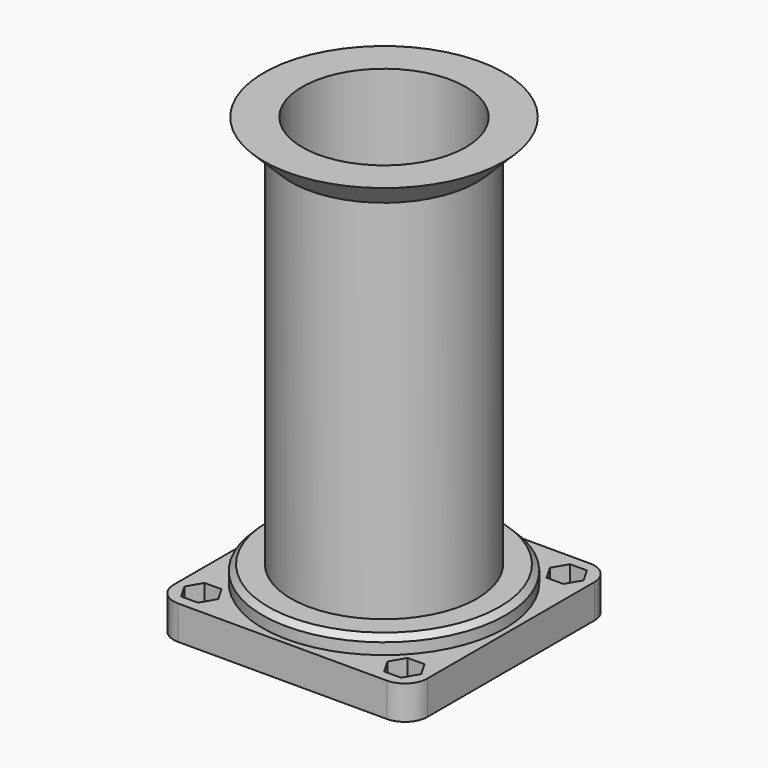
from build123d import *

# Parameters (mm, degrees)
F0_W         = 45
F0_H         = 45
F0_R         = 1.7
F1_DEPTH     = 6
F2_R         = 1.7
F3_DEPTH     = 3
F4_R         = 4
F5_R         = 21.5
F6_DEPTH     = 3
F7_SIZE      = 1
F8_R         = 16.5
F9_DEPTH     = 65
F10_R        = 21.5
F11_DEPTH    = 4.8
F12_S5_R     = 16.5
F12_T6_DEPTH = 32
F13_R        = 14.5
F14_DEPTH    = 100


# Not quite as in the source:
# - a fillet or chamfer that OpenCascade refuses, or shapes differently, is made with other operations: its cross-section is extruded or revolved along the edge and cut away or added


with BuildPart() as f1:
    # F0 (on Top) → F1 (new body)
    with BuildSketch(Plane.XY):
        with Locations((7.8061202839, 6.3967237547)):
            Rectangle(F0_W, F0_H)
        with Locations((-10.1938797161, -11.6032762453)):
            Circle(F0_R, mode=Mode.SUBTRACT)
        with Locations((25.8061202839, -11.6032762453)):
            Circle(F0_R, mode=Mode.SUBTRACT)
        with Locations((-10.1938797161, 24.3967237547)):
            Circle(F0_R, mode=Mode.SUBTRACT)
        with Locations((25.8061202839, 24.3967237547)):
            Circle(F0_R, mode=Mode.SUBTRACT)
    extrude(amount=F1_DEPTH)

    # F2 (on face) → F3 (cut)
    with BuildSketch(Plane.XY.offset(6)):
        Polygon((-11.694990416, 21.7967237547), (-8.6927690162, 21.7967237547), (-7.1916583163, 24.3967237547), (-8.6927690162, 26.9967237547), (-11.694990416, 26.9967237547), (-13.1961011159, 24.3967237547), align=None)
        with Locations((-10.1938797161, 24.3967237547)):
            Circle(F2_R, mode=Mode.SUBTRACT)
        Polygon((24.305009584, 21.7967237547), (27.3072309838, 21.7967237547), (28.8083416837, 24.3967237547), (27.3072309838, 26.9967237547), (24.305009584, 26.9967237547), (22.8038988841, 24.3967237547), align=None)
        with Locations((25.8061202839, 24.3967237547)):
            Circle(F2_R, mode=Mode.SUBTRACT)
        Polygon((-8.6927690162, -9.0032762453), (-11.694990416, -9.0032762453), (-13.1961011159, -11.6032762453), (-11.694990416, -14.2032762453), (-8.6927690162, -14.2032762453), (-7.1916583163, -11.6032762453), align=None)
        with Locations((-10.1938797161, -11.6032762453)):
            Circle(F2_R, mode=Mode.SUBTRACT)
        Polygon((27.3072309838, -9.0032762453), (24.305009584, -9.0032762453), (22.8038988841, -11.6032762453), (24.305009584, -14.2032762453), (27.3072309838, -14.2032762453), (28.8083416837, -11.6032762453), align=None)
        with Locations((25.8061202839, -11.6032762453)):
            Circle(F2_R, mode=Mode.SUBTRACT)
    extrude(amount=-F3_DEPTH, mode=Mode.SUBTRACT)

    # F4
    f4_edges = [f1.edges().sort_by_distance(p)[0] for p in [
        (-14.69388, 28.896724, 3),
        (30.30612, 28.896724, 3),
        (30.30612, -16.103276, 3),
        (-14.69388, -16.103276, 3),
    ]]
    fillet(f4_edges, radius=F4_R)

    # F5 (on face) → F6 (join)
    with BuildSketch(Plane.XY.offset(6)):
        with Locations((7.8061202839, 6.3967237547)):
            Circle(F5_R)
    extrude(amount=F6_DEPTH)

    # F7
    f7_edges = [f1.edges().sort_by_distance(p)[0] for p in [
        (-13.69388, 6.396724, 9),
    ]]
    chamfer(f7_edges, length=F7_SIZE)

    # F8 (on face) → F9 (join)
    with BuildSketch(Plane.XY.offset(9)):
        with Locations((7.8061202839, 6.3967237547)):
            Circle(F8_R)
    extrude(amount=F9_DEPTH)

    # F10 (on face) → F11 (join)
    with BuildSketch(Plane.XY.offset(74)):
        with Locations((7.8061202839, 6.3967237547)):
            Circle(F10_R)
    extrude(amount=F11_DEPTH)

    # F12: chamfer of 5 on 1 edges, made by hand


with BuildPart() as f12_tool2:
    # F12_s3 → F12_t4 (revolve)
    with BuildSketch(Plane.XZ.offset(-6.3967237547)):
        Polygon((29.3061202839, 79), (24.3061202839, 74), (29.3061202839, 74), align=None)
    revolve(axis=Axis((7.8061202839, 6.3967237547, 74), (0, 0, 1)))

    # F12_s5 → F12_t6 (cut, symmetric)
    with BuildSketch(Plane.XY.offset(76.5)):
        with Locations((7.8061202839, 6.3967237547)):
            Circle(F12_S5_R)
    extrude(amount=F12_T6_DEPTH, both=True, mode=Mode.SUBTRACT)


with BuildPart() as f1_1:
    add(f1.part)

    # F12_t1: cut F12_tool2
    add(f12_tool2.part, mode=Mode.SUBTRACT)

    # F13 (on face) → F14 (cut)
    with BuildSketch(Plane.XY.offset(78.8)):
        with Locations((7.8061202839, 6.3967237547)):
            Circle(F13_R)
    extrude(amount=-F14_DEPTH, mode=Mode.SUBTRACT)


solid = f1_1.part
